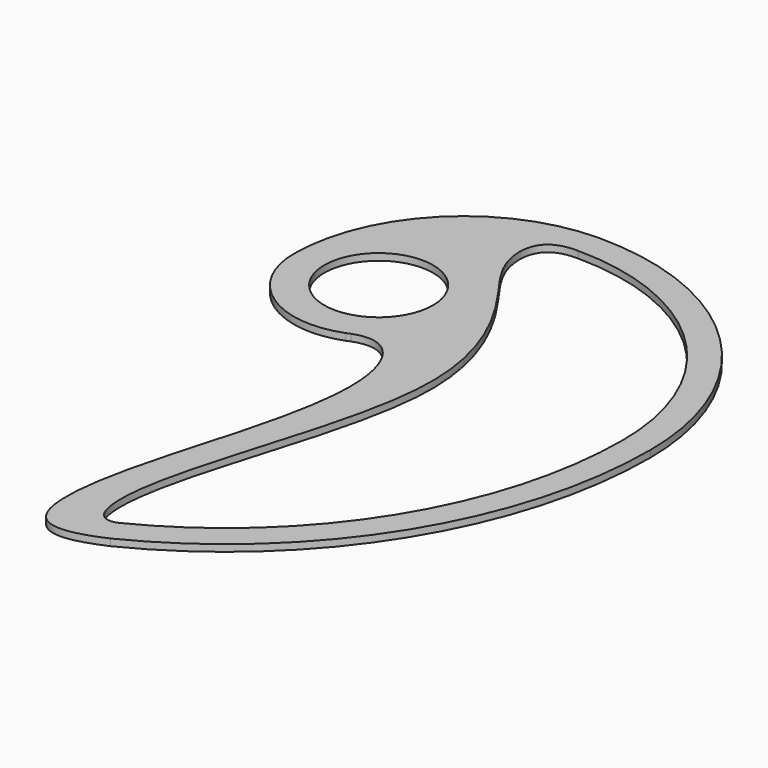
from build123d import *

# Parameters (mm, degrees)
F0_R     = 40
F1_DEPTH = 5


with BuildPart() as f1:
    # F0 (on Top) → F1 (new body)
    with BuildSketch(Plane.XY):
        with BuildLine():
            ThreePointArc((62.5, 125), (-25.8883476483, 88.3883476483), (-62.5, 0))
            ThreePointArc((-62.5, 0), (-35.3718816601, -51.5274682847), (22.4625596104, -58.3239523331))
            add(Edge.make_bspline(
                [(22.4625596104, -58.3239523331), (23.4338104217, -57.8834943524), (24.3880812611, -57.4889863625), (25.3254434787, -57.1390576804)],
                knots=[0, 0, 0, 0, 0.0078086947, 0.0078086947, 0.0078086947, 0.0078086947], degree=3))
            add(Edge.make_bspline(
                [(25.3254434787, -57.1390576804), (49.0548698892, -48.2805750634), (85.7849542145, -104.4302855165), (25.8955771825, -258.4521048553), (19.1129913649, -356.0221825551), (54.6846931143, -352.1963888275), (76.5954563413, -342.3369239847)],
                knots=[0.0078086947, 0.0078086947, 0.0078086947, 0.0078086947, 0.2054866489, 0.5709414839, 0.8143834536, 1, 1, 1, 1], degree=3))
            ThreePointArc((76.5954563413, -342.3369239847), (203.1346928647, -227.1039487578), (250, -62.5))
            ThreePointArc((250, -62.5), (195.0825214725, 70.0825214725), (62.5, 125))
        make_face()
        Circle(F0_R, mode=Mode.SUBTRACT)
        with BuildLine():
            ThreePointArc((62.5, 105), (180.9403858487, 55.9403858487), (230, -62.5))
            ThreePointArc((230, -62.5), (186.1340725214, -216.5692960373), (67.6933471355, -324.4273608496))
            add(Edge.make_bspline(
                [(67.6933471355, -324.4273608496), (52.1590419089, -329.9769233014), (40.1870983678, -267.654203975), (126.5199671093, -78.3907724821), (66.3352424241, 30.3993926076), (32.7769246578, 68.4207557353), (37.4844764475, 105.4154422107), (62.5, 105)],
                knots=[0, 0, 0, 0, 0.1437363374, 0.4686085678, 0.7052388709, 0.8608320173, 1, 1, 1, 1], degree=3))
        make_face(mode=Mode.SUBTRACT)
    extrude(amount=F1_DEPTH)


solid = f1.part
